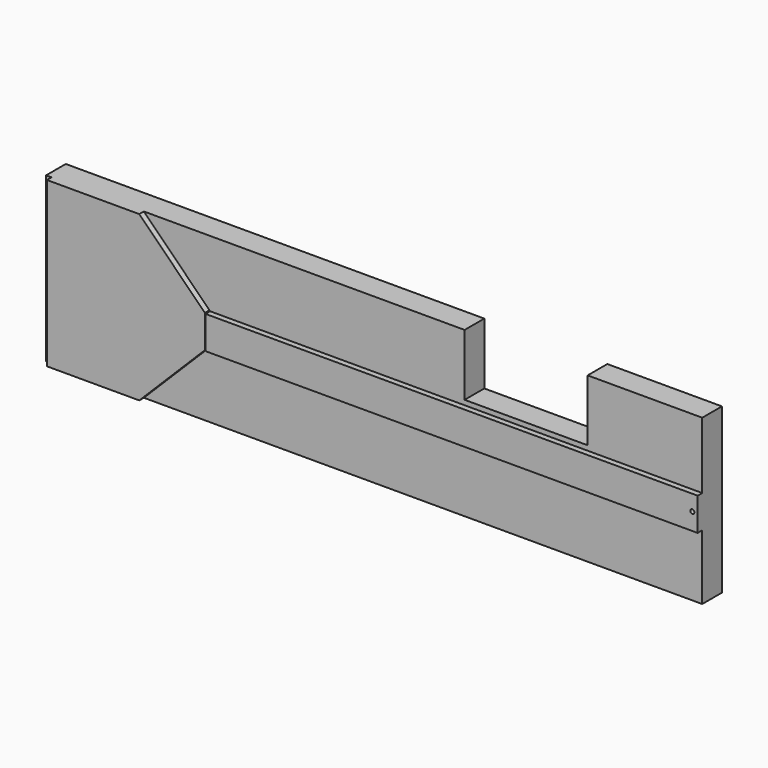
from build123d import *

# Parameters (mm, degrees)
F0_R        = 0.635
F1_DEPTH    = 3.81
F2_T        = 2.54
F2_T3_DEPTH = 12.7
F3_W        = 152.4
F3_H        = 10.16
F3_R        = 0.635
F4_DEPTH    = 1.778
F5_W        = 48.9099100232
F5_H        = 50.8
F6_DEPTH    = 1.778
F7_SIZE     = 20.32


# Not quite as in the source:
# - a shell that OpenCascade refuses in one call is made with other operations: the cavity is built on its own and cut out


with BuildPart() as f1:
    # F0 (on Front) → F1 (new body, symmetric)
    with BuildSketch(Plane.XZ):
        Polygon((101.6, -25.4), (101.6, 25.4), (66.1107632279, 25.4), (66.1107632279, 6.35), (28.0107632279, 6.35), (28.0107632279, 25.4), (-101.6, 25.4), (-101.6, -25.4), align=None)
        with Locations((99.9609604478, 0)):
            Circle(F0_R, mode=Mode.SUBTRACT)
        with Locations((-100.653603673, 3.1339845154)):
            Circle(F0_R, mode=Mode.SUBTRACT)
    extrude(amount=F1_DEPTH, both=True)

    # F2: shell of thickness 2.54, made by hand


with BuildPart() as f2_core1:
    # F2_t2: copy of F1
    add(f1.part)

    # the walls: a layer under each face that stays
    f2_faces = [f2_core1.faces().sort_by_distance(p)[0] for p in [
        (101.6, 0, 0),
        (0, 0, -25.4),
        (-101.6, 0, 0),
        (-36.794618386, 0, 25.4),
        (28.0107632279, 0, 15.875),
        (47.0607632279, 0, 6.35),
        (66.1107632279, 0, 15.875),
        (0, -3.81, 0),
        (-101.288603673, 0, 3.1339845154),
        (99.3259604478, 0, 0),
        (83.855381614, 0, 25.4),
    ]]
    thicken(f2_faces, amount=-F2_T, mode=Mode.SUBTRACT)

    # F2_s4 → F2_t3 (cut)
    with BuildSketch(Plane.XZ.offset(-6.35)):
        Polygon((28.0361632279, 6.3754), (25.4707632279, 6.35), (25.4707632279, 3.81), (28.0107632279, 3.81), align=None)
        Polygon((66.0853632279, 6.3754), (66.1107632279, 3.81), (68.6507632279, 3.81), (68.6507632279, 6.35), align=None)
    extrude(amount=F2_T3_DEPTH, mode=Mode.SUBTRACT)


with BuildPart() as f1_1:
    add(f1.part)

    # what is left inside the walls is the cavity
    f2_cavity = [f2_core1.part.solids().sort_by_distance(p)[0] for p in [
        (0, 3.7846, -7.62),
    ]]
    add(f2_cavity, mode=Mode.SUBTRACT)

    # F3 (on face) → F4 (join)
    with BuildSketch(Plane.XZ.offset(3.81)):
        with Locations((25.4, -0.2157475356)):
            Rectangle(F3_W, F3_H)
        with Locations((99.9609604478, 0)):
            Circle(F3_R, mode=Mode.SUBTRACT)
    extrude(amount=F4_DEPTH)

    # F5 (on face) → F6 (join)
    with BuildSketch(Plane.XZ.offset(3.81)):
        with Locations((-75.4546709359, 0)):
            Rectangle(F5_W, F5_H)
    extrude(amount=F6_DEPTH)

    # F7
    f7_edges = [f1_1.edges().sort_by_distance(p)[0] for p in [
        (-50.999716, -4.699, 25.4),
        (-50.999716, -4.699, -25.4),
    ]]
    chamfer(f7_edges, length=F7_SIZE)


solid = f1_1.part
